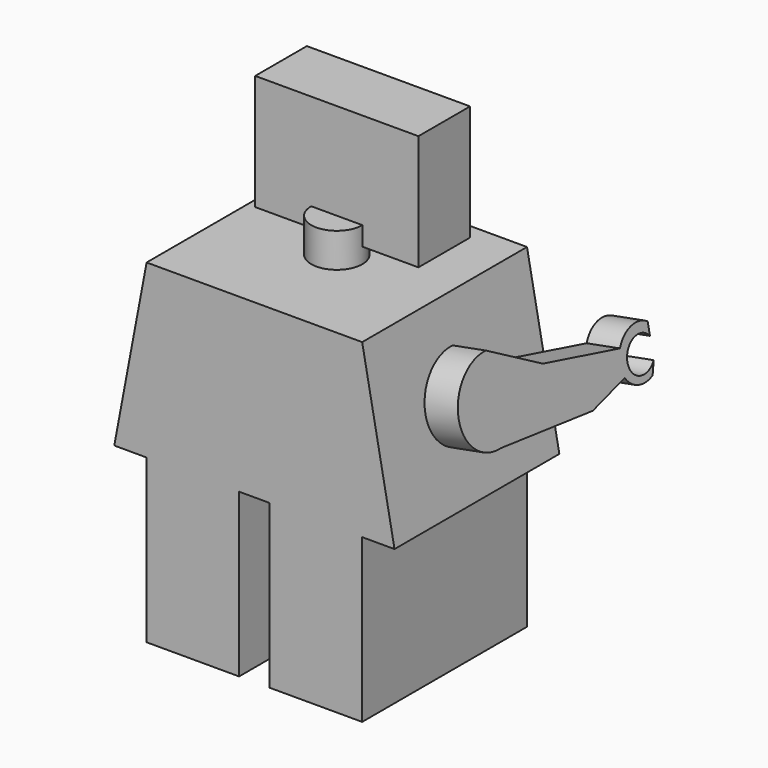
from build123d import *

# Parameters (mm, degrees)
F0_W     = 11.4046361996
F0_H     = 20.0534798205
F1_DEPTH = 12.7
F3_DEPTH = 4.17264
F5_R     = 3.1549889686
F6_DEPTH = 25.4
F7_W     = 10.0605683401
F7_H     = 14.2366550863
F8_DEPTH = 7.95975


with BuildPart() as f1:
    # F0 (on Front) → F1 (new body, symmetric)
    with BuildSketch(Plane.XZ):
        Polygon((-13.2875442505, 21.1651604623), (-17.2738078982, 0), (-13.2875442505, 0), (-1.8829080509, 0), (0, 0), (0, 21.1651604623), align=None)
        with Locations((-7.5852261507, -10.0267399102)):
            Rectangle(F0_W, F0_H)
        Polygon((13.2875442505, 21.1651604623), (0, 21.1651604623), (0, 0), (1.8829080509, 0), (13.2875442505, 0), (17.2738078982, 0), align=None)
        with Locations((7.5852261507, -10.0267399102)):
            Rectangle(F0_W, F0_H)
    extrude(amount=F1_DEPTH, both=True)

    # F2 (on face) → F3 (join)
    with BuildSketch(Plane(origin=(-16.6820575494, 0, 3.1419123751), x_dir=(0, -1, 0), z_dir=(-0.982722195, 0, 0.1850867027))):
        with BuildLine():
            Line((-13.796438463, 1.4029195299), (0, 2.9041063972))
            ThreePointArc((0, 2.9041063972), (5.3533335924, 7.9779976513), (0, 13.0518889055))
            Line((0, 13.0518889055), (-7.7627915889, 8.660916239))
            Line((-7.7627915889, 8.660916239), (-19.0092052332, 5.8628071696))
            ThreePointArc((-19.0092052332, 5.8628071696), (-18.616808085, 4.3270320221), (-19.026460126, 2.7957691345))
            Line((-19.026460126, 2.7957691345), (-13.796438463, 1.4029195299))
        make_face()
        with BuildLine():
            ThreePointArc((-23.0272375047, 1.4844691614), (-20.7737198496, 1.3678224494), (-19.026460126, 2.7957691345))
            ThreePointArc((-19.026460126, 2.7957691345), (-18.616808085, 4.3270320221), (-19.0092052332, 5.8628071696))
            ThreePointArc((-19.0092052332, 5.8628071696), (-21.0317417116, 7.3939934823), (-23.5248878598, 6.9255838171))
            Line((-23.5248878598, 6.9255838171), (-23.5248878598, 5.4076067172))
            ThreePointArc((-23.5248878598, 5.4076067172), (-19.7584909862, 4.1445688112), (-23.5248878598, 2.8815309051))
            Line((-23.5248878598, 2.8815309051), (-23.0272375047, 1.4844691614))
        make_face()
    extrude(amount=F3_DEPTH)

    # F4: F1 across plane


with BuildPart() as f1_1:
    add(f1.part)
    add(f1.part.mirror(Plane.YZ))

    # F5 (on Top) → F6 (join)
    with BuildSketch(Plane.XY):
        Circle(F5_R)
    extrude(amount=F6_DEPTH)

    # F7 (on Front) → F8 (join)
    with BuildSketch(Plane.XZ):
        with Locations((5.0302841701, 30.1817078143)):
            Rectangle(F7_W, F7_H)
        with Locations((-5.0302841701, 30.1817078143)):
            Rectangle(F7_W, F7_H)
    extrude(amount=-F8_DEPTH)


solid = f1_1.part
